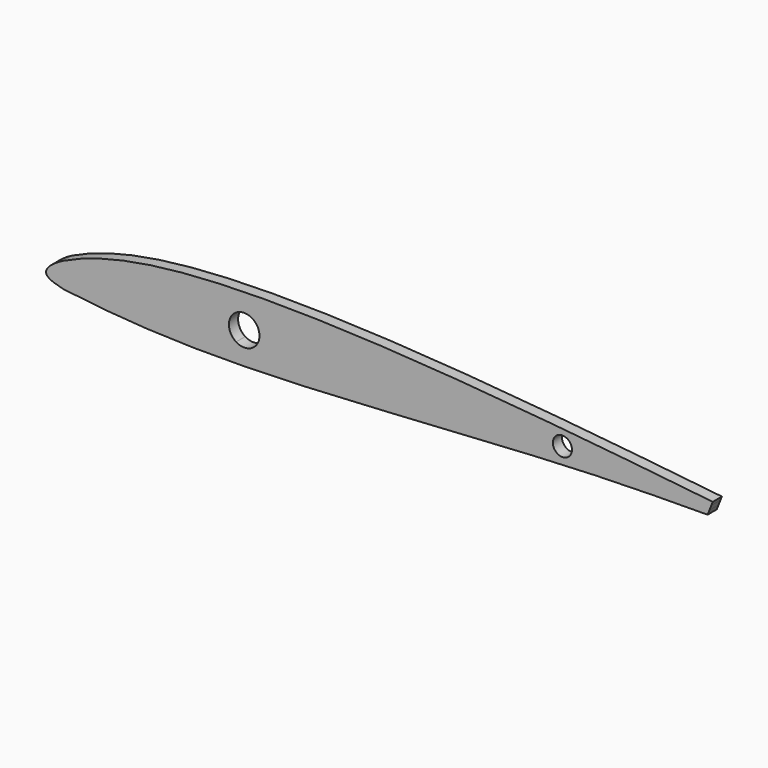
from build123d import *

# Parameters (mm, degrees)
F2_DEPTH = 3
F1_R     = 2.5
F3_DEPTH = 3
F4_DEPTH = 3


with BuildPart() as f2:
    # F0 (on Front) → F2 (new body)
    with BuildSketch(Plane.XZ):
        with BuildLine():
            add(Edge.make_bspline(
                [(-96.9805282175, -0.8100506688), (-84.7869920978, 5.1468541776), (-43.2313518226, 10.3846705605), (26.8477938201, 4.0208678603), (73.1462007926, -1.0427900778)],
                knots=[0, 0, 0, 0, 0.374886421, 0.9004696716, 0.9004696716, 0.9004696716, 0.9004696716], degree=3))
            add(Edge.make_bspline(
                [(-97.5447368223, -7.1186651935), (-99.939251346, -6.5508492693), (-102.885147974, -5.168950634), (-100.0067471137, -2.3789404522), (-96.9805282175, -0.8100506688)],
                knots=[0.0564585679, 0.0564585679, 0.0564585679, 0.0564585679, 0.4847104148, 1, 1, 1, 1], degree=3))
            add(Edge.make_bspline(
                [(-96.5428845142, -7.3406707446), (-96.8949965543, -7.2673488468), (-97.22905608, -7.1935231869), (-97.5447368223, -7.1186651935)],
                knots=[0, 0, 0, 0, 0.0564585679, 0.0564585679, 0.0564585679, 0.0564585679], degree=3))
            add(Edge.make_bspline(
                [(-96.5428845142, -7.3406707446), (-80.7020161693, -9.4302402111), (-44.2471235075, -11.1181020976), (27.9226364637, -4.7767282079), (62.4434148738, -4.5021877215), (71.7967184236, -4.4503783305)],
                knots=[0, 0, 0, 0, 0.2987594418, 0.6837410955, 0.8381168975, 0.8381168975, 0.8381168975, 0.8381168975], degree=3))
            Line((71.7967184236, -4.4503783305), (72.2670713195, -3.2626866351))
            add(Edge.make_bspline(
                [(-97.3825784566, -6.0471531808), (-82.3468325761, -8.841713568), (-44.2551066449, -8.6286827794), (32.5707299039, -3.8332069517), (63.1103828262, -3.2710139005), (72.2670713195, -3.2626866351)],
                knots=[0, 0, 0, 0, 0.3131273629, 0.7122131732, 0.9019797674, 0.9019797674, 0.9019797674, 0.9019797674], degree=3))
            add(Edge.make_bspline(
                [(-97.3825784566, -6.0471531808), (-98.6588937786, -5.8946130057), (-100.1661659123, -5.1778479876), (-99.9138553768, -4.2244412327), (-99.8196757147, -4.047003109)],
                knots=[0, 0, 0, 0, 0.4440177242, 0.5425000514, 0.5425000514, 0.5425000514, 0.5425000514], degree=3))
            add(Edge.make_bspline(
                [(-99.8196757147, -4.047003109), (-99.3821638101, -3.2227137691), (-97.9006497107, -2.3042858417), (-96.3385477662, -1.6362179573)],
                knots=[0.5425000514, 0.5425000514, 0.5425000514, 0.5425000514, 1, 1, 1, 1], degree=3))
            add(Edge.make_bspline(
                [(-96.3385477662, -1.6362179573), (-85.7442874691, 3.2900694446), (-41.4192830911, 9.6956733525), (28.5693195485, 2.5855104747), (72.7689680214, -1.9953434339)],
                knots=[0, 0, 0, 0, 0.384923117, 0.9441251659, 0.9441251659, 0.9441251659, 0.9441251659], degree=3))
            Line((72.7689680214, -1.9953434339), (73.1462007926, -1.0427900778))
        make_face()
        with BuildLine():
            add(Edge.make_bspline(
                [(-96.5428845142, -7.3406707446), (-96.8949965543, -7.2673488468), (-97.22905608, -7.1935231869), (-97.5447368223, -7.1186651935)],
                knots=[0, 0, 0, 0, 0.0564585679, 0.0564585679, 0.0564585679, 0.0564585679], degree=3))
            ThreePointArc((-97.5447368223, -7.1186651935), (-97.052492706, -7.2688477084), (-96.5428845142, -7.3406707446))
        make_face()
        with BuildLine():
            Line((72.2670713195, -3.2626866351), (72.7689680214, -1.9953434339))
            add(Edge.make_bspline(
                [(-96.3385477662, -1.6362179573), (-85.7442874691, 3.2900694446), (-41.4192830911, 9.6956733525), (28.5693195485, 2.5855104747), (72.7689680214, -1.9953434339)],
                knots=[0, 0, 0, 0, 0.384923117, 0.9441251659, 0.9441251659, 0.9441251659, 0.9441251659], degree=3))
            add(Edge.make_bspline(
                [(-99.8196757147, -4.047003109), (-99.3821638101, -3.2227137691), (-97.9006497107, -2.3042858417), (-96.3385477662, -1.6362179573)],
                knots=[0.5425000514, 0.5425000514, 0.5425000514, 0.5425000514, 1, 1, 1, 1], degree=3))
            add(Edge.make_bspline(
                [(-97.3825784566, -6.0471531808), (-98.6588937786, -5.8946130057), (-100.1661659123, -5.1778479876), (-99.9138553768, -4.2244412327), (-99.8196757147, -4.047003109)],
                knots=[0, 0, 0, 0, 0.4440177242, 0.5425000514, 0.5425000514, 0.5425000514, 0.5425000514], degree=3))
            add(Edge.make_bspline(
                [(-97.3825784566, -6.0471531808), (-82.3468325761, -8.841713568), (-44.2551066449, -8.6286827794), (32.5707299039, -3.8332069517), (63.1103828262, -3.2710139005), (72.2670713195, -3.2626866351)],
                knots=[0, 0, 0, 0, 0.3131273629, 0.7122131732, 0.9019797674, 0.9019797674, 0.9019797674, 0.9019797674], degree=3))
        make_face()
    extrude(amount=F2_DEPTH)


with BuildPart() as f2b:
    # F1 (on Front) → F2, piece 2 (new body)
    with BuildSketch(Plane.XZ):
        with BuildLine():
            ThreePointArc((-45.542362095, -1.3708024857), (-51.4789804014, 2.1291274472), (-51.6671168627, -4.7598166753))
            Line((-51.6671168627, -4.7598166753), (-47.385046135, -4.7391830831))
            ThreePointArc((-47.385046135, -4.7391830831), (-46.0331411102, -3.2905337378), (-45.542362095, -1.3708024857))
        make_face()
        with BuildLine():
            Line((-47.385046135, -4.7391830831), (-51.6671168627, -4.7598166753))
            ThreePointArc((-51.6671168627, -4.7598166753), (-49.523087913, -5.3707560487), (-47.385046135, -4.7391830831))
        make_face()
    extrude(amount=F2_DEPTH)


with BuildPart() as f2c:
    # F1 (on Front) → F2, piece 3 (new body)
    with BuildSketch(Plane.XZ):
        with Locations((33.7789729238, -1.0305350879)):
            Circle(F1_R)
    extrude(amount=F2_DEPTH)


with BuildPart() as f3_tool:
    # F3 (cut): a face of the model
    f3_faces = [f2b.part.faces().sort_by_distance(p)[0] for p in [
        (-49.542362095, -3, -1.3708024857),
    ]]
    extrude(f3_faces, amount=-F3_DEPTH)


with BuildPart() as f2_1:
    add(f2.part)

    # F3: cut by f3_tool
    add(f3_tool.part, mode=Mode.SUBTRACT)


with BuildPart() as f2b_1:
    add(f2b.part)

    # F3: cut by f3_tool
    add(f3_tool.part, mode=Mode.SUBTRACT)


with BuildPart() as f4_tool:
    # F4 (cut): a face of the model
    f4_faces = [f2c.part.faces().sort_by_distance(p)[0] for p in [
        (33.7789729238, -3, -1.0305350879),
    ]]
    extrude(f4_faces, amount=-F4_DEPTH)


with BuildPart() as f2_2:
    add(f2_1.part)

    # F4: cut by f4_tool
    add(f4_tool.part, mode=Mode.SUBTRACT)


with BuildPart() as f2c_1:
    add(f2c.part)

    # F4: cut by f4_tool
    add(f4_tool.part, mode=Mode.SUBTRACT)


solid = f2_2.part
